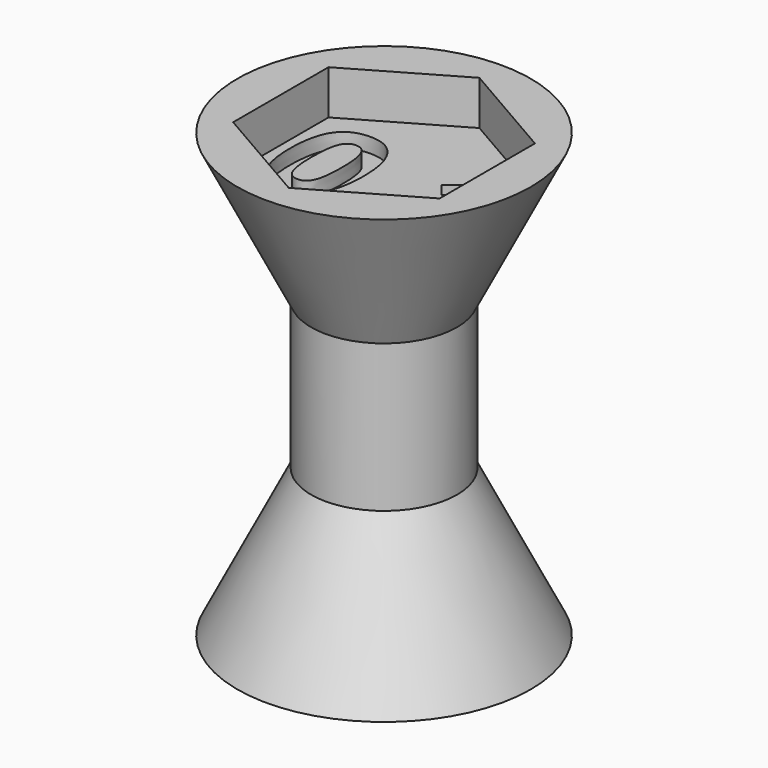
from build123d import *

# Parameters (mm, degrees)
F3_DEPTH     = 3
F4_TEXT_SIZE = 10.1151441231
F5_DEPTH     = 1


# Not quite as in the source:
# - Text() gives the source's letters only with a copy of the font that has no kerning and outlines rounded to 1/6400 em; it was checked with that copy


with BuildPart() as f1:
    # F0 (on Front) → F1 (revolve)
    with BuildSketch(Plane.XZ):
        Polygon((9.95, 15.0315666614), (0, 15.0315666614), (0, -14.9684333386), (9.95, -14.9684333386), (4.95, -4.9684333386), (4.95, 5.0315666614), align=None)
    revolve(axis=Axis((0, 0, 0.0315666614), (0, 0, -1)))

    # F2 (on face) → F3 (cut)
    with BuildSketch(Plane.XY.offset(15.0315666614)):
        Polygon((7, 4.0414518843), (0, 8.0829037687), (-7, 4.0414518843), (-7, -4.0414518843), (0, -8.0829037687), (7, -4.0414518843), align=None)
    extrude(amount=-F3_DEPTH, mode=Mode.SUBTRACT)

    # F4 (on face) → F5 (cut)
    with BuildSketch(Plane.XY.offset(12.0315666614)):
        with Locations((-6.7463269827, -3.6414518843)):
            Text('0.1', F4_TEXT_SIZE, font='Open Sans', font_style=FontStyle.BOLD, text_align=(TextAlign.LEFT, TextAlign.BOTTOM))
    extrude(amount=-F5_DEPTH, mode=Mode.SUBTRACT)


solid = f1.part
